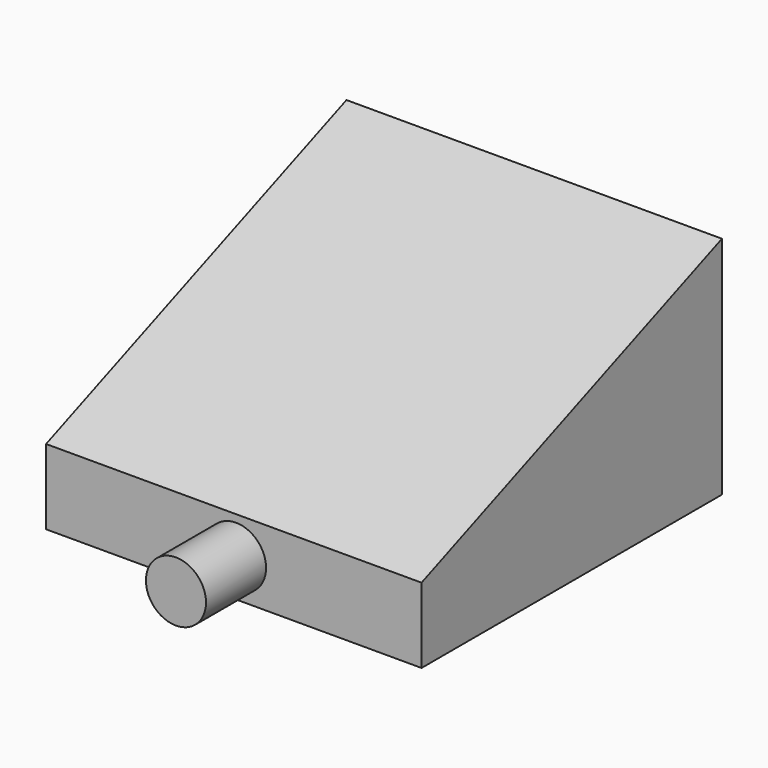
from build123d import *

# Parameters (mm, degrees)
F0_W     = 114.1541988105
F0_H     = 25.4
F1_DEPTH = 127
F2_R     = 10.16
F3_DEPTH = 25.4


# Not quite as in the source:
# - a feature names something its author has since deleted; it is built from what else it names


with BuildPart() as f1:
    # F0 (on Right) → F1 (new body)
    with BuildSketch(Plane.YZ):
        Polygon((127, 63.5), (0, 12.7), (12.8458011895, 12.7), (127, 12.7), align=None)
        with Locations((69.9229005948, 0)):
            Rectangle(F0_W, F0_H)
        Polygon((12.8458011895, 12.7), (0, 12.7), (0, 0), (0, -12.7), (12.8458011895, -12.7), align=None)
    extrude(amount=F1_DEPTH)

    # F2 (on face) → F3 (join)
    with BuildSketch(Plane.XZ):
        with Locations((64.2495304346, 0)):
            Circle(F2_R)
    extrude(amount=F3_DEPTH)


solid = f1.part
